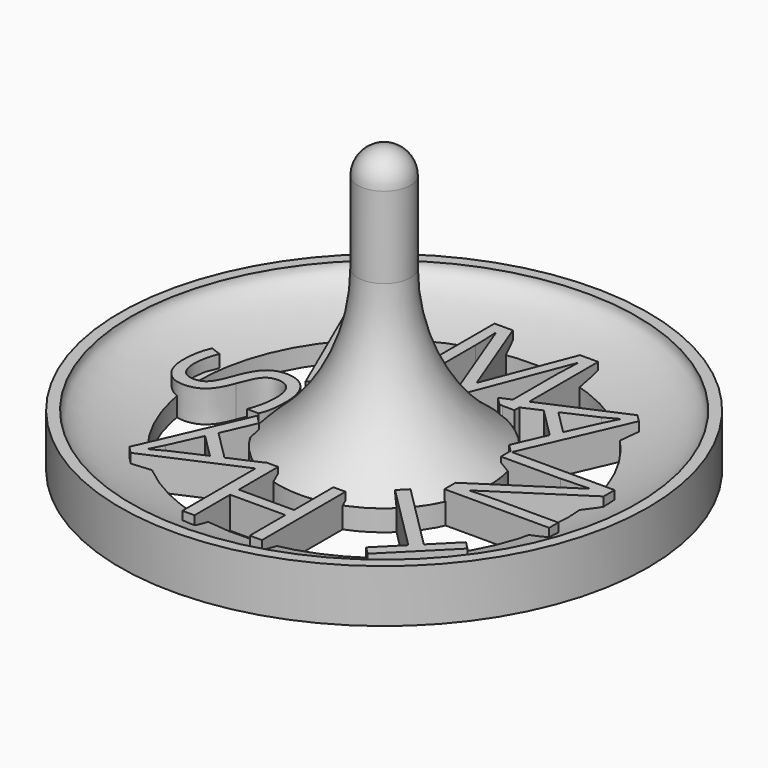
from build123d import *

# Parameters (mm, degrees)
F0_R         = 25
F0_R_2       = 17.5
F1_DEPTH     = 5
F4_R         = 10
F5_DEPTH     = 2
F6_TEXT_SIZE = 13.8888888889
F7_DEPTH     = 3
F10_R        = 3
F11_DEPTH    = 6


# Not quite as in the source:
# - Text() gives the source's letters only with a copy of the font that has no kerning and outlines rounded to 1/6400 em; it was checked with that copy


with BuildPart() as f1:
    # F0 (on Top) → F1 (new body)
    with BuildSketch(Plane.XY):
        Circle(F0_R)
        Circle(F0_R_2, mode=Mode.SUBTRACT)
    extrude(amount=F1_DEPTH)

    # F2 (on Front) → F3 (revolve, cut)
    with BuildSketch(Plane.XZ):
        with BuildLine():
            add(Edge.make_bspline(
                [(0, 9.5248220199), (-23.9752158523, 9.5248220199), (-23.9752158523, 4.9227378331)],
                knots=[4.7123889804, 4.7123889804, 4.7123889804, 6.2831853072, 6.2831853072, 6.2831853072], degree=2, weights=[1, 0.7071067812, 1]))
            add(Edge.make_bspline(
                [(-23.9752158523, 4.9227378331), (-23.9752158523, 0.3206536463), (0, 0.3206536463)],
                knots=[0, 0, 0, 1.5707963268, 1.5707963268, 1.5707963268], degree=2, weights=[1, 0.7071067812, 1]))
            Line((0, 0.3206536463), (0, 9.5248220199))
        make_face()
    revolve(axis=Axis((0, 0, 4.9227378331), (0, 0, -1)), mode=Mode.SUBTRACT)


with BuildPart() as f5:
    # F4 (on Top) → F5 (new body)
    with BuildSketch(Plane.XY):
        Circle(F4_R)
    extrude(amount=F5_DEPTH)


with BuildPart() as f7:
    # F6 (on Top) → F7 (new body)
    with BuildSketch(Plane.XY):
        with Locations(Location((-9, -3.9290364583), (0, 0, 90))):
            Text('S', F6_TEXT_SIZE, font='Open Sans', text_align=(TextAlign.LEFT, TextAlign.BOTTOM))
        Polygon((-7.5217563137, 9.6654806481), (-4.4189570264, 8.3089650349), (-3.7279220614, 9), (-4.6788194444, 9), (-4.6788194444, 9.6354632594), (-13.3728807856, 13.4357961025), (-14.0588111918, 12.7498656963), (-9.789776762, 2.9381452993), (-8.9642050427, 3.7637170187), (-10.3314622953, 6.8557746665), align=None)
        with BuildLine():
            Line((-11.4976974379, 11.5023009977), (-8.5084526251, 10.1457853845))
            Line((-8.5084526251, 10.1457853845), (-10.7764730734, 7.8777649361))
            Line((-10.7764730734, 7.8777649361), (-12.125316087, 10.8746823486))
            add(Edge.make_bspline(
                [(-12.8342642921, 12.1882314039), (-12.4797901896, 11.6219935518), (-12.125316087, 10.8746823486)],
                knots=[0, 0, 0, 1, 1, 1], degree=2))
            add(Edge.make_bspline(
                [(-11.4976974379, 11.5023009977), (-12.0685388498, 11.7570313052), (-12.8342642921, 12.1882314039)],
                knots=[0, 0, 0, 1, 1, 1], degree=2))
        make_face(mode=Mode.SUBTRACT)
        Polygon((-4.6788194444, 9), (-3.7279220614, 9), (-3.61328125, 9.1146408114), (-3.61328125, 9.1696970729), (-4.6788194444, 9.6354632594), align=None)
        Polygon((-3.61328125, 9.1146408114), (-3.7279220614, 9), (-3.61328125, 9), align=None)
        Polygon((-3.61328125, 9.1696970729), (-3.61328125, 9.1146408114), (-3.574971068, 9.1529509934), align=None)
        with BuildLine():
            Line((-4.6788194444, 9.6354632594), (-3.61328125, 9.1696970729))
            Line((-3.61328125, 9.1696970729), (-3.61328125, 15.3064236111))
            add(Edge.make_bspline(
                [(-3.7087673611, 17.7890625), (-3.61328125, 16.7452256944), (-3.61328125, 15.3064236111)],
                knots=[0, 0, 0, 1, 1, 1], degree=2))
            Line((-3.7087673611, 17.7890625), (-3.6545138889, 17.7890625))
            Line((-3.6545138889, 17.7890625), (-0.2907986111, 9))
            Line((-0.2907986111, 9), (0.6380208333, 9))
            Line((0.6380208333, 9), (4.0299479167, 17.7760416667))
            Line((4.0299479167, 17.7760416667), (4.0842013889, 17.7760416667))
            add(Edge.make_bspline(
                [(3.9887152778, 15.3888888889), (3.9887152778, 16.4869791667), (4.0842013889, 17.7760416667)],
                knots=[0, 0, 0, 1, 1, 1], degree=2))
            Line((3.9887152778, 15.3888888889), (3.9887152778, 10.246874929))
            Line((3.9887152778, 10.246874929), (5.1410590278, 10.7482543961))
            Line((5.1410590278, 10.7482543961), (5.1410590278, 18.9153645833))
            Line((5.1410590278, 18.9153645833), (3.41796875, 18.9153645833))
            Line((3.41796875, 18.9153645833), (0.2517361111, 10.7361111111))
            Line((0.2517361111, 10.7361111111), (0.1974826389, 10.7361111111))
            Line((0.1974826389, 10.7361111111), (-2.9427083333, 18.9153645833))
            Line((-2.9427083333, 18.9153645833), (-4.6788194444, 18.9153645833))
            Line((-4.6788194444, 18.9153645833), (-4.6788194444, 9.6354632594))
        make_face()
        Polygon((5.1410590278, 9.5732431221), (5.1410590278, 10.7482543961), (3.9887152778, 10.246874929), (3.9887152778, 9.063695588), align=None)
        Polygon((12.7498656963, 14.0588111918), (5.1410590278, 10.7482543961), (5.1410590278, 9.5732431221), (6.8557746665, 10.3314622953), (9.6654806481, 7.5217563137), (8.3089650349, 4.4189570264), (9.0864290058, 3.6414930556), (9.1820289679, 3.6414930556), (13.4357961025, 13.3728807856), align=None)
        with BuildLine():
            Line((11.5023009977, 11.4976974379), (10.1457853845, 8.5084526251))
            Line((10.1457853845, 8.5084526251), (7.8777649361, 10.7764730734))
            Line((7.8777649361, 10.7764730734), (10.8746823486, 12.125316087))
            add(Edge.make_bspline(
                [(12.1882314039, 12.8342642921), (11.6219935518, 12.4797901896), (10.8746823486, 12.125316087)],
                knots=[0, 0, 0, 1, 1, 1], degree=2))
            add(Edge.make_bspline(
                [(11.5023009977, 11.4976974379), (11.7570313052, 12.0685388498), (12.1882314039, 12.8342642921)],
                knots=[0, 0, 0, 1, 1, 1], degree=2))
        make_face(mode=Mode.SUBTRACT)
        Polygon((3.9887152778, 9.063695588), (3.9887152778, 10.246874929), (2.9381452993, 9.789776762), (3.7637170187, 8.9642050427), align=None)
        Polygon((5.1410590278, 9), (5.1410590278, 9.5732431221), (3.9887152778, 9.063695588), (3.9887152778, 9), align=None)
        with BuildLine():
            Line((18.9153645833, 3.6414930556), (9.1820289679, 3.6414930556))
            Line((9.1820289679, 3.6414930556), (9.1529509934, 3.574971068))
            Line((9.1529509934, 3.574971068), (9.0864290058, 3.6414930556))
            Line((9.0864290058, 3.6414930556), (9, 3.6414930556))
            Line((9, 3.6414930556), (9, 2.5759548611))
            Line((9, 2.5759548611), (14.6358506944, 2.5759548611))
            add(Edge.make_bspline(
                [(17.3203125, 2.6844618056), (15.85546875, 2.5759548611), (14.6358506944, 2.5759548611)],
                knots=[0, 0, 0, 1, 1, 1], degree=2))
            Line((17.3203125, 2.6844618056), (17.3203125, 2.6302083333))
            Line((17.3203125, 2.6302083333), (9, -2.7886284722))
            Line((9, -2.7886284722), (9, -4.1037326389))
            Line((9, -4.1037326389), (18.9153645833, -4.1037326389))
            Line((18.9153645833, -4.1037326389), (18.9153645833, -3.0251736111))
            Line((18.9153645833, -3.0251736111), (13.2252604167, -3.0251736111))
            add(Edge.make_bspline(
                [(11.8038194444, -3.0598958333), (12.7977430556, -3.0121527778), (13.2252604167, -3.0251736111)],
                knots=[0, 0, 0, 1, 1, 1], degree=2))
            add(Edge.make_bspline(
                [(10.6276041667, -3.1206597222), (10.8098958333, -3.1076388889), (11.8038194444, -3.0598958333)],
                knots=[0, 0, 0, 1, 1, 1], degree=2))
            Line((10.6276041667, -3.1206597222), (10.6276041667, -3.06640625))
            Line((10.6276041667, -3.06640625), (18.9153645833, 2.3394097222))
            Line((18.9153645833, 2.3394097222), (18.9153645833, 3.6414930556))
        make_face()
        Polygon((9.1529509934, 3.574971068), (9.1820289679, 3.6414930556), (9.0864290058, 3.6414930556), align=None)
        with Locations(Location((9.3532058435, -3.3747162179), (0, 0, -135))):
            Text('T', F6_TEXT_SIZE, font='Open Sans', text_align=(TextAlign.LEFT, TextAlign.BOTTOM))
        Polygon((-3.855782823, -9.0049150336), (-3.9837670275, -9.0050779353), (-3.9836952428, -9.0614758107), align=None)
        Polygon((-3.7637170187, -8.9642050427), (-3.855782823, -9.0049150336), (-3.7231758135, -9.0047462478), align=None)
        Polygon((-3.7231758135, -9.0047462478), (-3.855782823, -9.0049150336), (-3.9836952428, -9.0614758107), (-3.9821900489, -10.244035832), (-2.9381452993, -9.789776762), align=None)
        Polygon((-3.9821900489, -10.244035832), (-3.9836952428, -9.0614758107), (-6.8557746665, -10.3314622953), (-9.6654806481, -7.5217563137), (-8.3089650349, -4.4189570264), (-9.1529509934, -3.574971068), (-13.4357961025, -13.3728807856), (-12.7498656963, -14.0588111918), align=None)
        with BuildLine():
            Line((-11.5023009977, -11.4976974379), (-10.1457853845, -8.5084526251))
            Line((-10.1457853845, -8.5084526251), (-7.8777649361, -10.7764730734))
            Line((-7.8777649361, -10.7764730734), (-10.8746823486, -12.125316087))
            add(Edge.make_bspline(
                [(-12.1882314039, -12.8342642921), (-11.6219935518, -12.4797901896), (-10.8746823486, -12.125316087)],
                knots=[0, 0, 0, 1, 1, 1], degree=2))
            add(Edge.make_bspline(
                [(-11.5023009977, -11.4976974379), (-11.7570313052, -12.0685388498), (-12.1882314039, -12.8342642921)],
                knots=[0, 0, 0, 1, 1, 1], degree=2))
        make_face(mode=Mode.SUBTRACT)
        Polygon((-2.831424211, -9.0036112026), (-3.7231758135, -9.0047462478), (-2.9381452993, -9.789776762), (-3.9821900489, -10.244035832), (-3.9711464974, -18.9204344867), (-2.8188036808, -18.9189677541), (-2.8241734139, -14.7002211714), (2.3993466603, -14.6935725358), (2.4047163935, -18.9123191185), (3.55705921, -18.9108523858), (3.5444386799, -8.9954958344), (2.3920958633, -8.996962567), (2.3980346114, -13.6627573986), (-2.8254854629, -13.6694060342), align=None)
    extrude(amount=F7_DEPTH)


with BuildPart() as f9:
    # F8 (on Front) → F9 (revolve)
    with BuildSketch(Plane.XZ):
        with BuildLine():
            Line((0, 24.5401822031), (0, 27.0401822031))
            ThreePointArc((0, 27.0401822031), (-1.767766953, 26.307949156), (-2.5, 24.5401822031))
            Line((-2.5, 24.5401822031), (0, 24.5401822031))
        make_face()
        with BuildLine():
            ThreePointArc((-2.5, 24.5401822031), (-1.767766953, 22.7724152501), (0, 22.0401822031))
            Line((0, 22.0401822031), (0, 24.5401822031))
            Line((0, 24.5401822031), (-2.5, 24.5401822031))
        make_face()
        with BuildLine():
            Line((0, 16.8360350719), (0, 22.0401822031))
            ThreePointArc((0, 22.0401822031), (-1.767766953, 22.7724152501), (-2.5, 24.5401822031))
            Line((-2.5, 24.5401822031), (-2.5, 16.8360350719))
            Line((-2.5, 16.8360350719), (0, 16.8360350719))
        make_face()
        with BuildLine():
            Line((0, 2), (0, 16.8360350719))
            Line((0, 16.8360350719), (-2.5, 16.8360350719))
            ThreePointArc((-2.5, 16.8360350719), (-4.4815626295, 8.5240266405), (-10, 2))
            Line((-10, 2), (0, 2))
        make_face()
    revolve(axis=Axis((0, 0, 9.4180175359), (0, 0, -1)))


with BuildPart() as f11_tool:
    # F10 (on Top) → F11 (new body)
    with BuildSketch(Plane.XY):
        Circle(F10_R)
    extrude(amount=F11_DEPTH)


with BuildPart() as f5_1:
    add(f5.part)

    # F11: cut by f11_tool
    add(f11_tool.part, mode=Mode.SUBTRACT)


with BuildPart() as f9_1:
    add(f9.part)

    # F11: cut by f11_tool
    add(f11_tool.part, mode=Mode.SUBTRACT)


solid = Compound([f1.part, f7.part, f5_1.part, f9_1.part])
